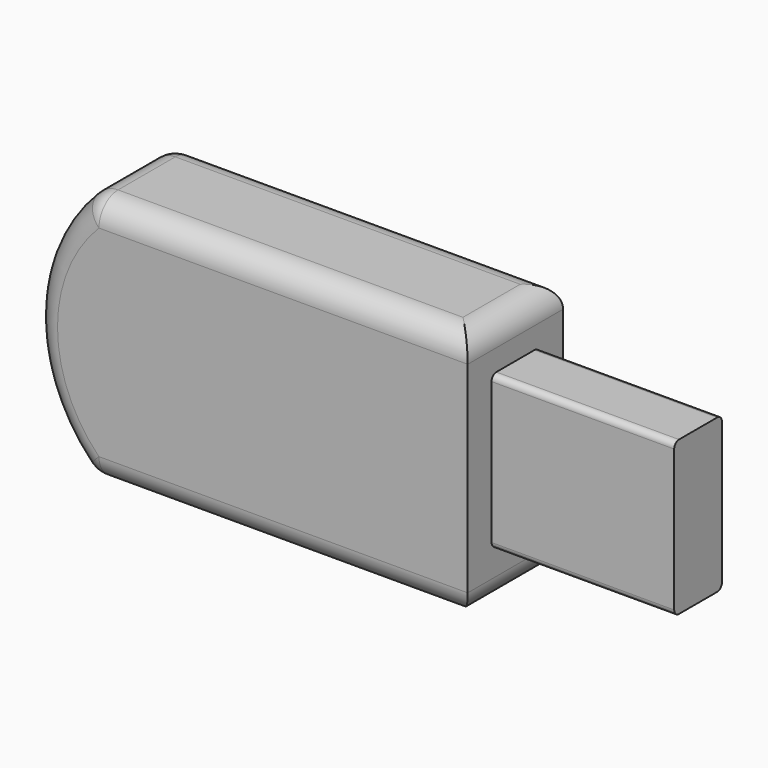
from build123d import *

# Parameters (mm, degrees)
F2_DEPTH = 12.7
F1_W     = 38.9029346406
F1_H     = 32.7060050331
F3_DEPTH = 6.35
F4_R     = 5.08
F5_R     = 1.27


# Not quite as in the source:
# - two fillets or chamfers of one size are made in one step
# - a feature names something its author has since deleted; it is built from what else it names


with BuildPart() as f2:
    # F0 (on Front) → F2 (new body, symmetric)
    with BuildSketch(Plane.XZ):
        with BuildLine():
            Line((-80.5600658059, -3.4427349456), (0, -3.4427349456))
            Line((0, -3.4427349456), (0, 49.5754186995))
            Line((0, 49.5754186995), (-80.5600658059, 49.5754186995))
            ThreePointArc((-80.5600658059, 49.5754186995), (-92.446291157, 23.066341877), (-80.5600658059, -3.4427349456))
        make_face()
    extrude(amount=F2_DEPTH, both=True)

    # F1 (on Front) → F3 (join, symmetric)
    with BuildSketch(Plane.XZ):
        with Locations((19.4514673203, 23.5827539582)):
            Rectangle(F1_W, F1_H)
    extrude(amount=F3_DEPTH, both=True)

    # F4
    f4_edges = [f2.edges().sort_by_distance(p)[0] for p in [
        (-40.280033, -12.7, -3.442735),
        (-40.280033, -12.7, 49.575419),
        (-40.280033, 12.7, -3.442735),
        (-40.280033, 12.7, 49.575419),
        (-92.446291, 12.7, 23.066342),
        (-80.560066, 0, -3.442735),
        (-92.446291, -12.7, 23.066342),
        (-80.560066, 0, 49.575419),
        (0, 0, -3.442735),
        (0, 0, 49.575419),
    ]]
    fillet(f4_edges, radius=F4_R)

    # F5
    f5_edges = [f2.edges().sort_by_distance(p)[0] for p in [
        (19.451467, -6.35, 39.935756),
        (19.451467, -6.35, 7.229751),
        (19.451467, 6.35, 39.935756),
        (19.451467, 6.35, 7.229751),
    ]]
    fillet(f5_edges, radius=F5_R)


solid = f2.part
